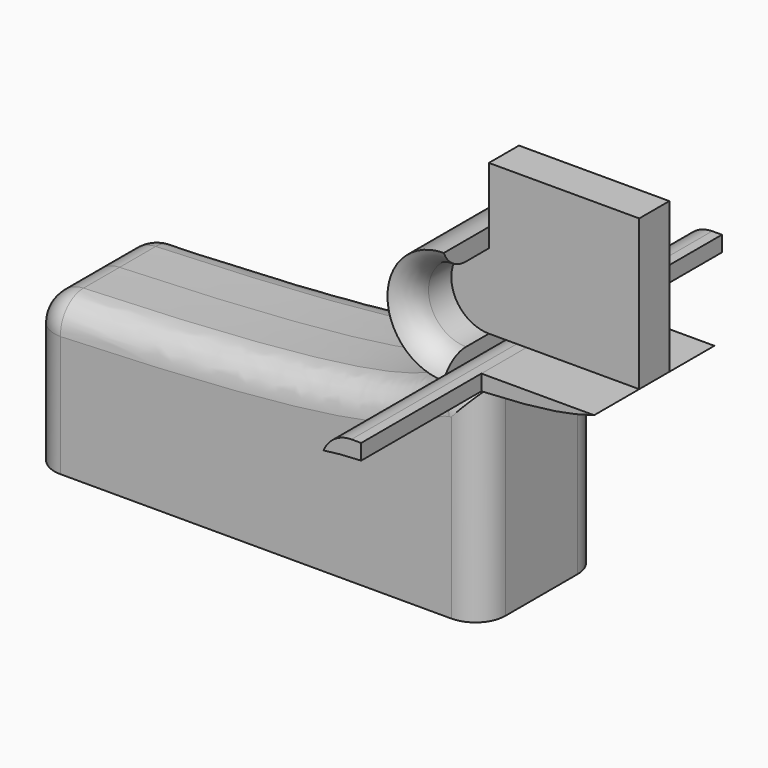
from build123d import *

# Parameters (mm, degrees)
F0_W          = 76.2
F0_H          = 25.4
F1_DEPTH      = 12.7
F2_DEPTH      = 38.1
F3_DEPTH      = 3.175
F4_F1_R       = 5.0796
F4_2_T2_ANGLE = 359.64
F4_2_T4_ANGLE = 359.64
F4_3_T1_DEPTH = 99.7464301965


# Not quite as in the source:
# - a fillet or chamfer that OpenCascade refuses, or shapes differently, is made with other operations: its cross-section is extruded or revolved along the edge and cut away or added
# - a fillet or chamfer is up to 0.001 mm smaller than in the source, because OpenCascade refuses the exact size


with BuildPart() as f1:
    # F0 (on Front) → F1 (new body, symmetric)
    with BuildSketch(Plane.XZ):
        Rectangle(F0_W, F0_H)
        with BuildLine():
            add(Edge.make_bspline(
                [(-38.1, 12.7), (32.512575388, 14.803212136), (23.5047876806, 20.7225713408), (31.75, 22.225)],
                knots=[0, 0, 0, 0, 0.6239927855, 0.6239927855, 0.6239927855, 0.6239927855], degree=3))
            Line((-38.1, 12.7), (38.1, 12.7))
            Line((38.1, 12.7), (38.1, 22.7704106553))
            add(Edge.make_bspline(
                [(31.75, 22.225), (33.3251560401, 22.5120222725), (35.5299749751, 22.6378449119), (38.1, 22.7704106553)],
                knots=[0.6239927855, 0.6239927855, 0.6239927855, 0.6239927855, 0.7431996618, 0.7431996618, 0.7431996618, 0.7431996618], degree=3))
        make_face()
    extrude(amount=F1_DEPTH, both=True)

    # F4: fillet of radius 5.08 on 8 edges, made by hand

    # F4_f1 (radius 5.08 in the source; OpenCascade refuses exactly that, so slightly less here)
    f4_f1_edges = [f1.edges().sort_by_distance(p)[0] for p in [
        (23.8023418909, -12.7, 18.7788236042),
        (23.8023418909, 12.7, 18.7788236042),
        (38.1, -12.7, 5.0352053276),
        (-38.1, 6.35, 12.7),
        (-38.1, -6.35, 12.7),
        (-38.1, 12.7, 0),
        (-38.1, -12.7, 0),
        (38.1, 12.7, 5.0352053276),
    ]]
    fillet(f4_f1_edges, radius=F4_F1_R)


with BuildPart() as f1b:
    # F0 (on Front) → F1, piece 2 (new body, symmetric)
    with BuildSketch(Plane.XZ):
        with BuildLine():
            ThreePointArc((31.75, 41.275), (22.225, 31.75), (31.75, 22.225))
            Line((31.75, 22.225), (31.75, 25.4))
            ThreePointArc((31.75, 25.4), (25.4, 31.75), (31.75, 38.1))
            Line((31.75, 38.1), (31.75, 41.275))
        make_face()
    extrude(amount=F1_DEPTH, both=True)

    # F4#2: fillet of radius 5.08 on 2 edges, made by hand

    # F4_2_s1 → F4_2_t2 (revolve, cut)
    with BuildSketch(Plane(origin=(0.1000582694, 0, 31.8494315515), x_dir=(0, 1, 0), z_dir=(0.0031415875, 0, 0.9999950652))):
        with BuildLine():
            ThreePointArc((7.9907139607, -38.0000979175), (10.8305202921, -38.8679844337), (12.7, -41.1750979175))
            Line((12.7, -41.1750979175), (12.7941857208, -41.1369979175))
            ThreePointArc((12.7941857208, -41.1369979175), (12.8016, -39.5875979175), (12.8016, -38.0000979175))
            Line((12.8016, -38.0000979175), (12.7, -37.8984979175))
            Line((12.7, -37.8984979175), (7.9907139607, -37.8984979175))
            Line((7.9907139607, -37.8984979175), (7.9907139607, -38.0000979175))
        make_face()
    revolve(axis=Axis((31.75, 12.7, 31.75), (0, 1, 0)), revolution_arc=F4_2_T2_ANGLE, mode=Mode.SUBTRACT)

    # F4_2_s3 → F4_2_t4 (revolve, cut)
    with BuildSketch(Plane(origin=(0.1000582694, 0, 31.8494315515), x_dir=(0, 1, 0), z_dir=(0.0031415875, 0, 0.9999950652))):
        with BuildLine():
            ThreePointArc((-7.9907139607, -38.0000979175), (-10.8305202921, -38.8679844337), (-12.7, -41.1750979175))
            Line((-12.7, -41.1750979175), (-12.7941857208, -41.1369979175))
            ThreePointArc((-12.7941857208, -41.1369979175), (-12.8016, -39.5875979175), (-12.8016, -38.0000979175))
            Line((-12.8016, -38.0000979175), (-12.7, -37.8984979175))
            Line((-12.7, -37.8984979175), (-7.9907139607, -37.8984979175))
            Line((-7.9907139607, -37.8984979175), (-7.9907139607, -38.0000979175))
        make_face()
    revolve(axis=Axis((31.75, -12.7, 31.75), (0, 1, 0)), revolution_arc=F4_2_T4_ANGLE, mode=Mode.SUBTRACT)


with BuildPart() as f1c:
    # F0 (on Front) → F1, piece 3 (new body, symmetric)
    with BuildSketch(Plane.XZ):
        with BuildLine():
            Line((38.1, 25.4), (38.1, 22.7704106553))
            add(Edge.make_bspline(
                [(38.1, 22.7704106553), (43.6364532308, 23.0559892123), (50.8677381583, 23.3728608571), (57.15, 25.4)],
                knots=[0.7431996618, 0.7431996618, 0.7431996618, 0.7431996618, 1, 1, 1, 1], degree=3))
            Line((57.15, 25.4), (38.1, 25.4))
        make_face()
    extrude(amount=F1_DEPTH, both=True)


with BuildPart() as f2:
    # F0 (on Front) → F2 (new body, symmetric)
    with BuildSketch(Plane.XZ):
        with BuildLine():
            Line((31.75, 25.4), (31.75, 22.225))
            add(Edge.make_bspline(
                [(31.75, 22.225), (33.3251560401, 22.5120222725), (35.5299749751, 22.6378449119), (38.1, 22.7704106553)],
                knots=[0.6239927855, 0.6239927855, 0.6239927855, 0.6239927855, 0.7431996618, 0.7431996618, 0.7431996618, 0.7431996618], degree=3))
            Line((38.1, 22.7704106553), (38.1, 25.4))
            Line((38.1, 25.4), (31.75, 25.4))
        make_face()
    extrude(amount=F2_DEPTH, both=True)

    # F4#3: fillet of radius 5.08 on 1 edges, made by hand

    # F4_3_s2 → F4_3_t1 (cut)
    with BuildSketch(Plane.XZ.offset(-49.8732150983)):
        with BuildLine():
            ThreePointArc((31.75, 22.225), (33.6194797079, 24.5321134838), (36.4592860393, 25.4))
            Line((36.4592860393, 25.4), (36.4592860393, 25.5016))
            Line((36.4592860393, 25.5016), (31.75, 25.5016))
            Line((31.75, 25.5016), (31.6484, 25.4))
            ThreePointArc((31.6484, 25.4), (31.6484, 23.8125), (31.6558142792, 22.2631))
            Line((31.6558142792, 22.2631), (31.75, 22.225))
        make_face()
    extrude(amount=F4_3_T1_DEPTH, mode=Mode.SUBTRACT)


with BuildPart() as f3:
    # F0 (on Front) → F3 (new body, symmetric)
    with BuildSketch(Plane.XZ):
        with BuildLine():
            Line((31.75, 50.8), (31.75, 41.275))
            Line((31.75, 41.275), (31.75, 38.1))
            ThreePointArc((31.75, 38.1), (25.4, 31.75), (31.75, 25.4))
            Line((31.75, 25.4), (38.1, 25.4))
            Line((38.1, 25.4), (57.15, 25.4))
            Line((57.15, 25.4), (57.15, 50.8))
            Line((57.15, 50.8), (31.75, 50.8))
        make_face()
    extrude(amount=F3_DEPTH, both=True)


solid = Compound([f1.part, f1b.part, f1c.part, f2.part, f3.part])
